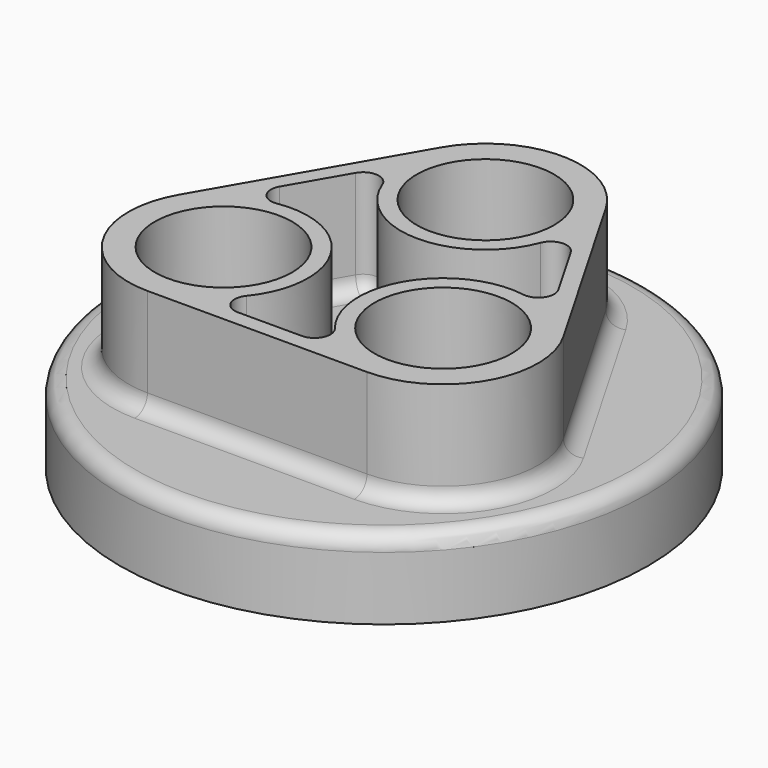
from build123d import *

# Parameters (mm, degrees)
F0_R         = 50
F1_DEPTH     = 15
F2_T         = -3
F4_DEPTH     = 20
F5_R         = 13
F6_DEPTH     = 35.001
F7_T         = 3
F7_T3_DEPTH  = 47.5692193817
F7_T5_DEPTH  = 47.5692193817
F7_T7_DEPTH  = 47.5692193817
F7_T10_ANGLE = 120.000000001
F7_T12_ANGLE = 120.000000001
F7_T14_ANGLE = 120.000000001
F8_R         = 3


# Not quite as in the source:
# - a shell that OpenCascade refuses in one call is made with other operations: the cavity is built on its own and cut out


with BuildPart() as f1:
    # F0 (on Top) → F1 (new body)
    with BuildSketch(Plane.XY):
        Circle(F0_R)
    extrude(amount=-F1_DEPTH)

    # F2
    f2_openings = [f1.faces().sort_by_distance(p)[0] for p in [
        (0, 0, -15),
    ]]
    offset(amount=F2_T, openings=f2_openings)

    # F3 (on face) → F4 (join)
    with BuildSketch(Plane.XY):
        with BuildLine():
            Line((36.3730669589, -3), (15.5884572681, 33))
            ThreePointArc((15.5884572681, 33), (0, 42), (-15.5884572681, 33))
            Line((-15.5884572681, 33), (-36.3730669589, -3))
            ThreePointArc((-36.3730669589, -3), (-36.3730669589, -21), (-20.7846096908, -30))
            Line((-20.7846096908, -30), (20.7846096908, -30))
            ThreePointArc((20.7846096908, -30), (36.3730669589, -21), (36.3730669589, -3))
        make_face()
    extrude(amount=F4_DEPTH)

    # F5 (on face) → F6 (cut, through all)
    with BuildSketch(Plane.XY.offset(20)):
        with Locations((0, 24)):
            Circle(F5_R)
        with Locations((-20.7846096908, -12)):
            Circle(F5_R)
        with Locations((20.7846096908, -12)):
            Circle(F5_R)
    extrude(amount=-F6_DEPTH, mode=Mode.SUBTRACT)

    # F7: shell of thickness 3, made by hand


with BuildPart() as f7_core1:
    # F7_t2: copy of F1
    add(f1.part)

    # the walls: a layer under each face that stays
    f7_faces = [f7_core1.faces().sort_by_distance(p)[0] for p in [
        (-50, 0, -7.5),
        (-33.3333333333, -33.3333333333, 0),
        (-33.3333333333, -33.3333333333, -15),
        (25.9807621135, 15, 10),
        (0, 42, 10),
        (-25.9807621135, 15, 10),
        (-36.3730669589, -21, 10),
        (0, -30, 10),
        (36.3730669589, -21, 10),
        (-47, 0, -9),
        (0, 0, -3),
        (-33.7846096908, -12, 8.5),
        (7.7846096908, -12, 8.5),
        (-13, 24, 8.5),
    ]]
    thicken(f7_faces, amount=-F7_T, mode=Mode.SUBTRACT)

    # F7_s4 → F7_t3 (cut)
    with BuildSketch(Plane(origin=(11.8923048454, -20.5980762114, 0), x_dir=(0, 0, 1), z_dir=(-0.5, 0.8660254038, 0))):
        Polygon((0.03, 30.03), (-3, 30), (-3, 27), (0, 27), align=None)
    extrude(amount=F7_T3_DEPTH, mode=Mode.SUBTRACT)

    # F7_s6 → F7_t5 (cut)
    with BuildSketch(Plane(origin=(11.8923048454, 20.5980762114, 0), x_dir=(0, 0, 1), z_dir=(-0.5, -0.8660254038, 0))):
        Polygon((0.03, 30.03), (-3, 30), (-3, 27), (0, 27), align=None)
    extrude(amount=F7_T5_DEPTH, mode=Mode.SUBTRACT)

    # F7_s8 → F7_t7 (cut)
    with BuildSketch(Plane.YZ.offset(-23.7846096908)):
        Polygon((-30.03, 0.03), (-30, -3), (-27, -3), (-27, 0), align=None)
    extrude(amount=F7_T7_DEPTH, mode=Mode.SUBTRACT)

    # F7_s9 → F7_t10 (revolve, cut)
    with BuildSketch(Plane(origin=(-10.3923048454, 18, 0), x_dir=(0, 0, 1), z_dir=(0.5, -0.8660254038, 0))):
        Polygon((0.03, -30.03), (-3, -30), (-3, -27), (0, -27), align=None)
    revolve(axis=Axis((0, 24, 0), (0, 0, 1)), revolution_arc=F7_T10_ANGLE, mode=Mode.SUBTRACT)

    # F7_s11 → F7_t12 (revolve, cut)
    with BuildSketch(Plane(origin=(-10.3923048454, -18, 0), x_dir=(0, 0, 1), z_dir=(0.5, 0.8660254038, 0))):
        Polygon((0.03, -30.03), (-3, -30), (-3, -27), (0, -27), align=None)
    revolve(axis=Axis((-20.7846096908, -12, 0), (0, 0, 1)), revolution_arc=F7_T12_ANGLE, mode=Mode.SUBTRACT)

    # F7_s13 → F7_t14 (revolve, cut)
    with BuildSketch(Plane.YZ.offset(20.7846096908)):
        Polygon((-30.03, 0.03), (-30, -3), (-27, -3), (-27, 0), align=None)
    revolve(axis=Axis((20.7846096908, -12, 0), (0, 0, 1)), revolution_arc=F7_T14_ANGLE, mode=Mode.SUBTRACT)

    # F7_s15 → F7_t16 (revolve, cut)
    with BuildSketch(Plane.XZ):
        Polygon((46.97, -3.03), (50, -3), (50, 0), (47, 0), align=None)
    revolve(axis=Axis((0, 0, -3), (0, 0, 1)), mode=Mode.SUBTRACT)


with BuildPart() as f1_1:
    add(f1.part)

    # what is left inside the walls is the cavity
    f7_cavity = [f7_core1.part.solids().sort_by_distance(p)[0] for p in [
        (6.902222, -3.985, 6.666667),
    ]]
    add(f7_cavity, mode=Mode.SUBTRACT)

    # F8
    f8_edges = [f1_1.edges().sort_by_distance(p)[0] for p in [
        (6.928203, -4, 0),
        (23.382686, 13.5, 0),
        (0, 8, 0),
        (-23.382686, 13.5, 0),
        (-6.928203, -4, 0),
        (0, -27, 0),
        (-25.980762, 15, 0),
        (-50, 0, 0),
        (25.980762, 15, 0),
        (0, 42, 0),
        (-36.373067, -21, 0),
        (0, -30, 0),
        (36.373067, -21, 0),
        (15.774263, 26.678175, 10),
        (30.991109, 0.321825, 10),
        (-15.774263, 26.678175, 10),
        (-30.991109, 0.321825, 10),
        (-15.216845, -27, 10),
        (15.216845, -27, 10),
    ]]
    fillet(f8_edges, radius=F8_R)


solid = f1_1.part
